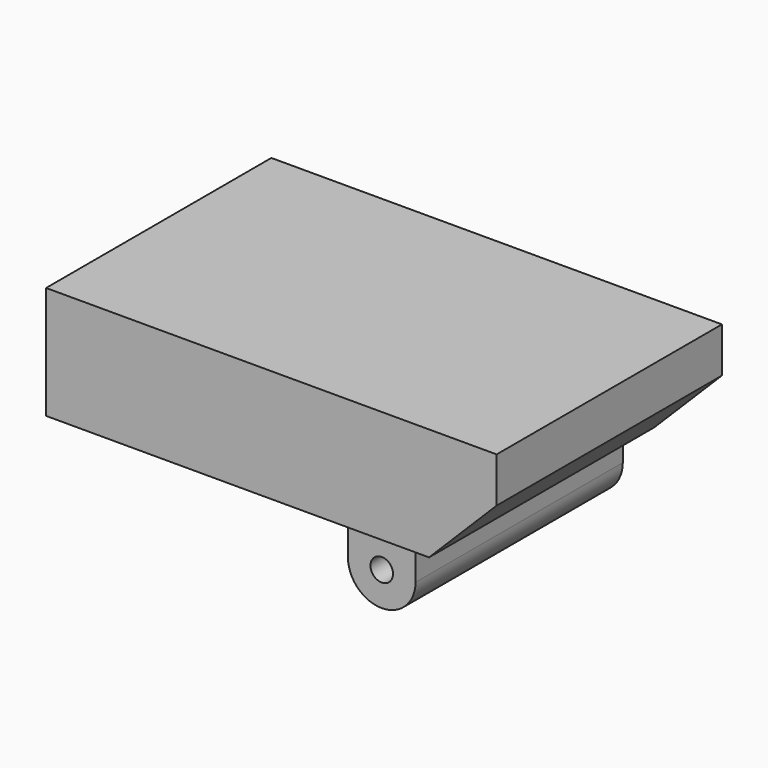
from build123d import *

# Parameters (mm, degrees)
F0_W      = 40
F0_H      = 25
F1_DEPTH  = 10
F2_W      = 6
F2_H      = 25
F3_DEPTH  = 6
F4_R      = 2.99999
F5_R      = 1
F6_DEPTH  = 30
F7_SIZE   = 6
F8_R      = 1
F9_DEPTH  = 1
F10_R     = 1
F11_DEPTH = 1


# Not quite as in the source:
# - a fillet or chamfer is up to 0.001 mm smaller than in the source, because OpenCascade refuses the exact size
# - ends of sketch curves that miss each other by under 0.0002 mm in the source are joined


with BuildPart() as f1:
    # F0 (on Top) → F1 (new body)
    with BuildSketch(Plane.XY):
        Rectangle(F0_W, F0_H)
    extrude(amount=F1_DEPTH)

    # F2 (on face) → F3 (join)
    with BuildSketch(Plane(origin=(0, 0, 0), x_dir=(1, 0, 0), z_dir=(0, 0, -1))):
        with Locations((9, 0)):
            Rectangle(F2_W, F2_H)
    extrude(amount=F3_DEPTH)

    # F4 (radius 3 in the source; OpenCascade refuses exactly that, so slightly less here)
    f4_edges = [f1.edges().sort_by_distance(p)[0] for p in [
        (6, 0, -6),
        (12, 0, -6),
    ]]
    fillet(f4_edges, radius=F4_R)

    # F5 (on face) → F6 (cut)
    with BuildSketch(Plane(origin=(0, 12.5, 0), x_dir=(-1, 0, 0), z_dir=(0, 1, 0))):
        with Locations((-9, -3)):
            Circle(F5_R)
    extrude(amount=-F6_DEPTH, mode=Mode.SUBTRACT)

    # F7
    f7_edges = [f1.edges().sort_by_distance(p)[0] for p in [
        (20, 0, 0),
    ]]
    chamfer(f7_edges, length=F7_SIZE)

    # F8 (on face) → F9 (cut)
    with BuildSketch(Plane(origin=(0, 12.5, 0), x_dir=(-1, 0, 0), z_dir=(0, 1, 0))):
        with BuildLine():
            Line((-6, -3.00001), (-6, 0))
            Line((-6, 0), (-12, 0))
            Line((-12, 0), (-12, -3.00001))
            ThreePointArc((-12, -3.00001), (-11.1213232725, -5.1213232725), (-9.00001, -6))
            ThreePointArc((-9.00001, -6), (-6.8786767275, -5.1213232725), (-6, -3.00001))
        make_face()
        with Locations((-9, -3)):
            Circle(F8_R, mode=Mode.SUBTRACT)
    extrude(amount=-F9_DEPTH, mode=Mode.SUBTRACT)

    # F10 (on face) → F11 (cut)
    with BuildSketch(Plane.XZ.offset(12.5)):
        with BuildLine():
            Line((12, 0), (6, 0))
            Line((6, 0), (6, -3.00001))
            ThreePointArc((6, -3.00001), (6.8786767275, -5.1213232725), (8.99999, -6))
            ThreePointArc((8.99999, -6), (11.1213232725, -5.1213232725), (12, -3.00001))
            Line((12, -3.00001), (12, 0))
        make_face()
        with Locations((9, -3)):
            Circle(F10_R, mode=Mode.SUBTRACT)
    extrude(amount=-F11_DEPTH, mode=Mode.SUBTRACT)


solid = f1.part
